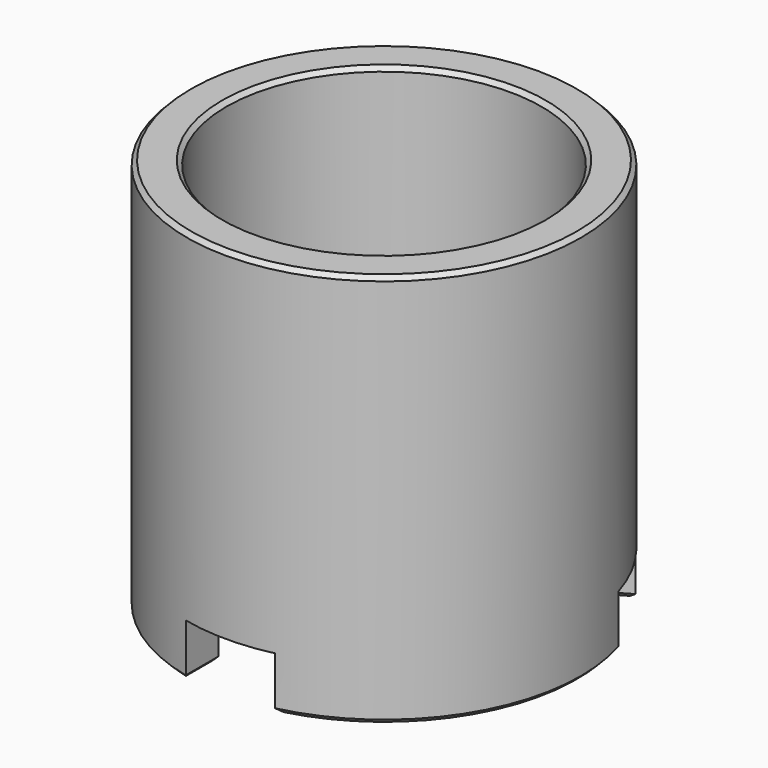
from build123d import *

# Parameters (mm, degrees)
F0_R     = 23.8125
F0_R_2   = 19.05
F1_DEPTH = 47.625
F2_W     = 10.795
F2_H     = 5.5431405764
F3_DEPTH = 6.35
F4_SIZE  = 0.508


with BuildPart() as f1:
    # F0 (on Top) → F1 (new body)
    with BuildSketch(Plane.XY):
        Circle(F0_R)
        Circle(F0_R_2, mode=Mode.SUBTRACT)
    extrude(amount=F1_DEPTH)

    # F2 (on face) → F3 (cut)
    with BuildSketch(Plane(origin=(0, 0, 0), x_dir=(1, 0, 0), z_dir=(0, 0, -1))):
        with Locations((0, 21.0409297118)):
            Rectangle(F2_W, F2_H)
        Polygon((-23.3209799276, -7.2318778831), (-17.9234799276, -16.5806221169), (-13.1229793717, -13.8090518287), (-18.5204793717, -4.4603075949), align=None)
        Polygon((17.9234799276, -16.5806221169), (23.3209799276, -7.2318778831), (18.5204793717, -4.4603075949), (13.1229793717, -13.8090518287), align=None)
    extrude(amount=-F3_DEPTH, mode=Mode.SUBTRACT)

    # F4
    f4_edges = [f1.edges().sort_by_distance(p)[0] for p in [
        (-23.8125, 0, 47.625),
        (-19.05, 0, 47.625),
        (-16.497784, -9.525, 0),
        (-20.62223, -11.90625, 0),
        (18.648902, -14.807214, 0),
        (15.259831, -11.403511, 0),
        (0, 19.05, 0),
        (0, 23.8125, 0),
        (-20.652356, 5.691147, 0),
        (-5.3975, -20.731039, 0),
        (5.3975, -20.731039, 0),
        (20.652356, 5.691147, 0),
        (15.254856, 15.039891, 0),
        (-15.254856, 15.039891, 0),
    ]]
    chamfer(f4_edges, length=F4_SIZE)


solid = f1.part
